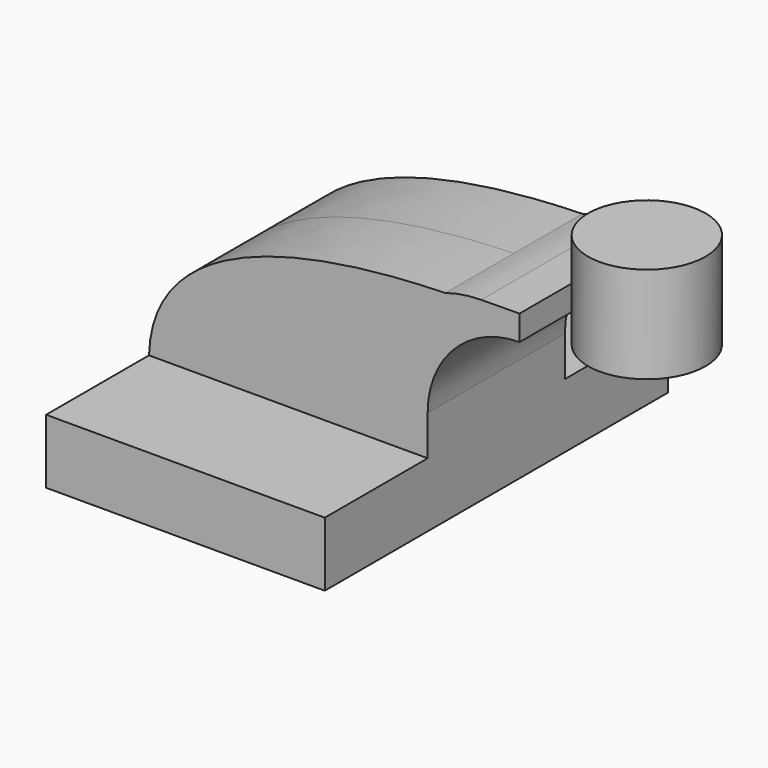
from build123d import *

# Parameters (mm, degrees)
F0_W     = 82.55
F0_H     = 19.05
F1_DEPTH = 63.5
F2_DEPTH = 25.4


# Not quite as in the source:
# - a feature names something its author has since deleted; it is built from what else it names


with BuildPart() as f1:
    # F0 (on Front) → F1 (new body, symmetric)
    with BuildSketch(Plane.XZ):
        Rectangle(F0_W, F0_H)
    extrude(amount=F1_DEPTH, both=True)

    # F0 (on Front) → F2 (join, symmetric)
    with BuildSketch(Plane.XZ):
        with BuildLine():
            add(Edge.make_bspline(
                [(-41.275, 9.525), (-40.358517319, 40.2696579695), (-3.6993576345, 52.9938253489), (46.4628638043, 54.3190308219)],
                knots=[0, 0, 0, 0, 98.5111056796, 98.5111056796, 98.5111056796, 98.5111056796], degree=3))
            Line((-41.275, 9.525), (41.275, 9.525))
            Line((41.275, 9.525), (41.275, 21.3973916233))
            ThreePointArc((41.275, 21.3973916233), (49.2381780267, 40.6567058334), (68.4772506356, 48.6686639759))
            Line((68.4772506356, 48.6686639759), (68.4772506356, 56.1067202576))
            Line((68.4772506356, 56.1067202576), (57.15, 55.9943579674))
            ThreePointArc((57.15, 55.9943579674), (51.741173854, 55.5729842221), (46.4628638043, 54.3190308219))
        make_face()
    extrude(amount=F2_DEPTH, both=True)

    # F0 (on Front) → F3 (revolve)
    with BuildSketch(Plane.XZ):
        Polygon((85.8719348907, 55.5244293195), (85.8719348907, 43.363083154), (103.2666191459, 43.363083154), (103.2666191459, 71.938083154), (85.8719348907, 71.938083154), align=None)
    revolve(axis=Axis((85.8719348907, 0, 57.650583154), (0, 0, 1)))


solid = f1.part
